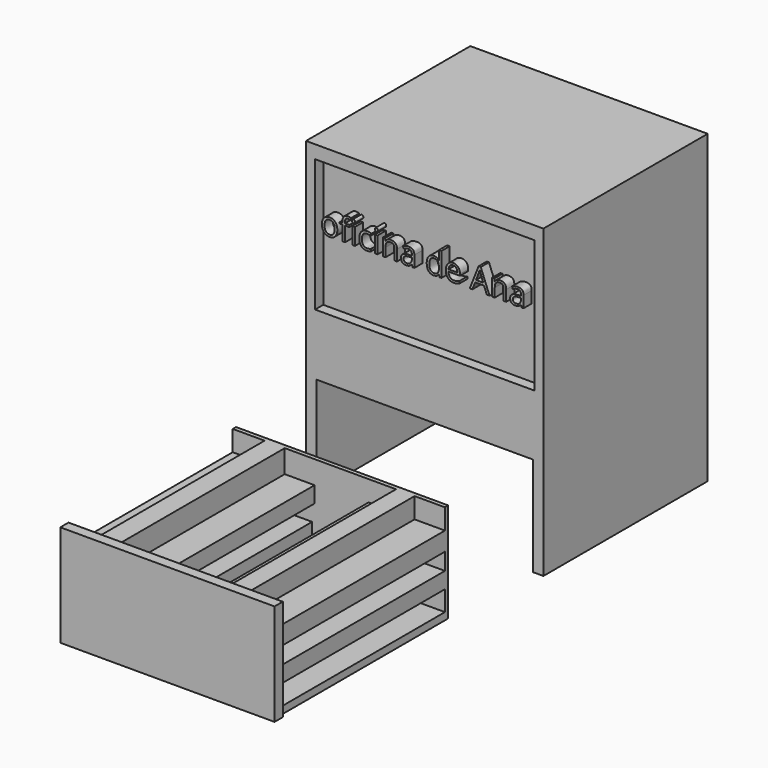
from build123d import *

# Parameters (mm, degrees)
F0_W         = 115.6037300825
F0_H         = 148.9373147488
F1_DEPTH     = 50
F2_W         = 106.7384555936
F2_H         = 64.4638563693
F3_DEPTH     = 5
F4_TEXT_SIZE = 15.2091254753
F5_DEPTH     = 5
F6_W         = 105.4206192493
F6_H         = 57.541107045
F7_DEPTH     = 100.001
F9_W         = 103.3242046833
F9_H         = 48.4730862081
F10_DEPTH    = 2
F12_DEPTH    = 100
F13_W        = 104.3178960681
F13_H        = 49.5067927986
F14_DEPTH    = 5


# Not quite as in the source:
# - Text() gives the source's letters only with a copy of the font that has no kerning and outlines rounded to 1/6400 em; it was checked with that copy


with BuildPart() as f1:
    # F0 (on Front) → F1 (new body, symmetric)
    with BuildSketch(Plane.XZ):
        Rectangle(F0_W, F0_H)
    extrude(amount=F1_DEPTH, both=True)

    # F2 (on face) → F3 (cut)
    with BuildSketch(Plane.XZ.offset(50)):
        with Locations((0, 35.8417694084)):
            Rectangle(F2_W, F2_H)
    extrude(amount=-F3_DEPTH, mode=Mode.SUBTRACT)

    # F4 (on face) → F5 (join)
    with BuildSketch(Plane.XZ.offset(45)):
        with Locations((-50.8889905815, 37.1632308385)):
            Text('oficina de Ana', F4_TEXT_SIZE, font='Open Sans', text_align=(TextAlign.LEFT, TextAlign.BOTTOM))
    extrude(amount=F5_DEPTH)

    # F6 (on face) → F7 (cut, through all)
    with BuildSketch(Plane.XZ.offset(50)):
        with Locations((0, -54.9678256579)):
            Rectangle(F6_W, F6_H)
    extrude(amount=-F7_DEPTH, mode=Mode.SUBTRACT)


with BuildPart() as f10:
    # F9 (on offset) → F10 (new body)
    with BuildSketch(Plane.XZ.offset(100)):
        with Locations((-0.2125911415, -50.1738954335)):
            Rectangle(F9_W, F9_H)
    extrude(amount=F10_DEPTH)

    # F11 (on face) → F12 (join)
    with BuildSketch(Plane.XZ.offset(102)):
        Polygon((-36.3718941808, -35.9169840813), (-51.8746934831, -35.9169840813), (-51.8746934831, -44.9488386512), (-35.5865173042, -44.9488386512), (-35.5865173042, -53.1953126192), (-51.8746934831, -53.1953126192), (-51.8746934831, -61.0490962863), (-35.5865173042, -61.0490962863), (-35.5865173042, -70.4736411572), (-51.8746934831, -70.4736411572), (-51.8746934831, -74.4104385376), (-13.2032250986, -74.4104385376), (-13.2032250986, -70.8663314581), (-26.5546627343, -70.8663314581), (-26.5546627343, -61.0490962863), (-13.2032250986, -61.0490962863), (-13.2032250986, -53.1953126192), (-27.3400396109, -53.1953126192), (-27.3400396109, -44.9488386512), (-12.025157921, -44.9488386512), (-12.025157921, -37.0950512588), (-26.5546627343, -37.0950512588), (-26.5546627343, -25.9373523295), (-36.3718941808, -25.9373523295), align=None)
        Polygon((51.4495112002, -44.9488386512), (51.4495112002, -35.9169840813), (36.6683155298, -35.9169840813), (36.6683155298, -25.9373523295), (27.6364590973, -25.9373523295), (27.6364590973, -35.9169840813), (14.2850270495, -35.9169840813), (14.2850270495, -44.9488386512), (26.0657034814, -44.9488386512), (26.0657034814, -53.1953126192), (13.8923386112, -53.1953126192), (13.8923386112, -61.0490962863), (26.4583937824, -61.0490962863), (26.4583937824, -70.8663314581), (13.8923386112, -70.8663314581), (13.8923386112, -74.4104385376), (51.4495112002, -74.4104385376), (51.4495112002, -70.8663314581), (36.6683155298, -70.8663314581), (36.6683155298, -61.0490962863), (51.4495112002, -61.0490962863), (51.4495112002, -53.1953126192), (36.6683155298, -53.1953126192), (36.6683155298, -44.9488386512), align=None)
    extrude(amount=F12_DEPTH)

    # F13 (on face) → F14 (join)
    with BuildSketch(Plane.XZ.offset(202)):
        with Locations((0.3179013729, -50.1738889143)):
            Rectangle(F13_W, F13_H)
    extrude(amount=F14_DEPTH)


solid = Compound([f1.part, f10.part])
